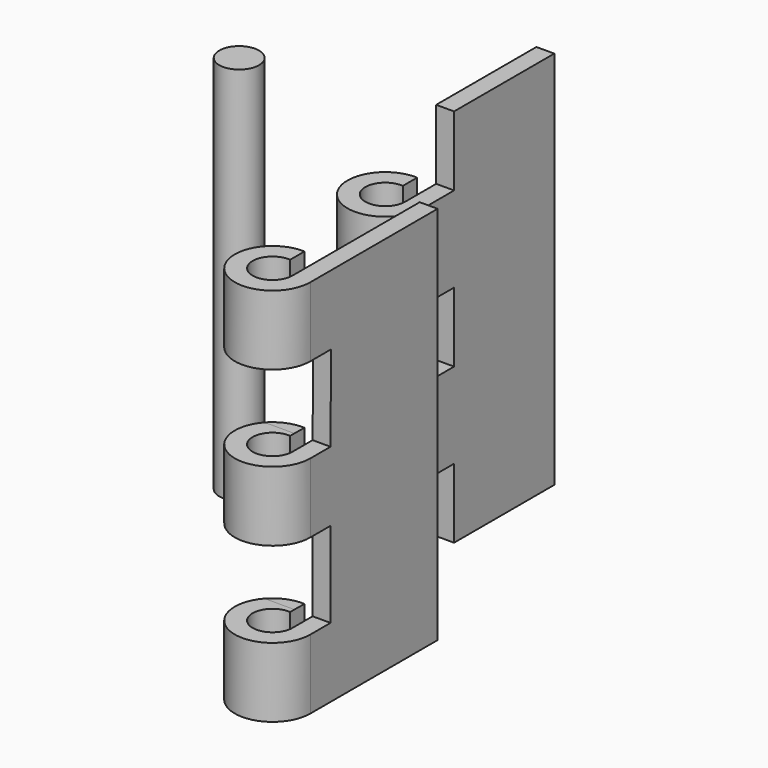
from build123d import *

# Parameters (mm, degrees)
F1_DEPTH = 19.1
F0_R     = 1
F2_W     = 2.3683065209
F2_H     = 4.3
F2_W_2   = 2.4908180475
F3_DEPTH = 15.1081433349
F4_W     = 2.6818022196
F4_H     = 3.5
F4_W_2   = 1.95
F4_W_3   = 2.4897197326
F5_DEPTH = 10.4387875527
F6_DEPTH = 19.9954353951


with BuildPart() as f1:
    # F0 (on Top) → F1 (new body)
    with BuildSketch(Plane.XY):
        with BuildLine():
            Line((10.7399763687, 0.6659325571), (10.7399763687, 8.6659325571))
            Line((10.7399763687, 8.6659325571), (9.8399763687, 8.6659325571))
            Line((9.8399763687, 8.6659325571), (9.8399763687, 0.6659325571))
            ThreePointArc((9.8399763687, 0.6659325571), (8.0998586216, -0.0112987509), (8.9243799683, 1.664056903))
            Line((8.9243799683, 1.664056903), (8.9243799683, 2.564056903))
            ThreePointArc((8.9243799683, 2.564056903), (7.466956551, -0.647390168), (10.7399763687, 0.6659325571))
        make_face()
    extrude(amount=F1_DEPTH)

    # F2 (on face) → F3 (cut, through all)
    with BuildSketch(Plane.YZ.offset(10.7399763687)):
        with Locations((-0.5182207033, 13.45)):
            Rectangle(F2_W, F2_H)
        Polygon((1.9321352011, 11.3), (1.9659325571, 15.6), (0.6659325571, 15.6), (0.6659325571, 11.3), align=None)
        with Locations((-0.5794764666, 5.65)):
            Rectangle(F2_W_2, F2_H)
        Polygon((1.9321352011, 7.8), (0.6659325571, 7.8), (0.6659325571, 3.5), (1.9321352011, 3.5), (1.9321352011, 7.4659469537), align=None)
    extrude(amount=-F3_DEPTH, mode=Mode.SUBTRACT)

    # F6 (cut, through all): faces of the model
    f6_faces = [f1.faces().sort_by_distance(p)[0] for p in [
        (8.1815308669, 1.9489752068, 13.4425351912),
        (8.1738825267, 1.9321352011, 5.65),
    ]]
    extrude(f6_faces, amount=-F6_DEPTH, dir=(0, -0.9999691128, 0.0078596075), mode=Mode.SUBTRACT)


with BuildPart() as f1b:
    # F0 (on Top) → F1, piece 2 (new body)
    with BuildSketch(Plane.XY):
        with BuildLine():
            Line((6.0706205865, 13.5883718793), (6.0706205865, 21.8383718793))
            Line((6.0706205865, 21.8383718793), (5.1706205865, 21.8383718793))
            Line((5.1706205865, 21.8383718793), (5.1706205865, 13.5883718793))
            ThreePointArc((5.1706205865, 13.5883718793), (3.4305028395, 12.9111405713), (4.2550241862, 14.5864962252))
            Line((4.2550241862, 14.5864962252), (4.2550241862, 15.4864962252))
            ThreePointArc((4.2550241862, 15.4864962252), (2.7976007689, 12.2750491542), (6.0706205865, 13.5883718793))
        make_face()
    extrude(amount=F1_DEPTH)

    # F4 (on face) → F5 (cut, through all)
    with BuildSketch(Plane.YZ.offset(6.0706205865)):
        with Locations((12.2474707695, 17.35)):
            Rectangle(F4_W, F4_H)
        with Locations((14.5633718793, 17.35)):
            Rectangle(F4_W_2, F4_H)
        Polygon((13.5883718793, 7.8), (13.5883718793, 11.3), (11.9571578597, 11.3), (10.8226276934, 11.3), (10.8226276934, 7.8), (11.9571578597, 7.8), align=None)
        Polygon((15.5383718793, 7.8), (15.5383718793, 11.3), (15.3883718793, 11.3), (13.5883718793, 11.3), (13.5883718793, 7.8), (15.3883718793, 7.8), align=None)
        with Locations((12.343512013, 1.75)):
            Rectangle(F4_W_3, F4_H)
        Polygon((15.3883718793, 0), (15.5383718793, 0), (15.5383718793, 3.5), (15.3883718793, 3.5), (13.5883718793, 3.5), (13.5883718793, 0), align=None)
    extrude(amount=-F5_DEPTH, mode=Mode.SUBTRACT)


with BuildPart() as f1c:
    # F0 (on Top) → F1, piece 3 (new body)
    with BuildSketch(Plane.XY):
        with Locations((-3.3671669662, 13.8250226155)):
            Circle(F0_R)
    extrude(amount=F1_DEPTH)


solid = Compound([f1.part, f1b.part, f1c.part])
